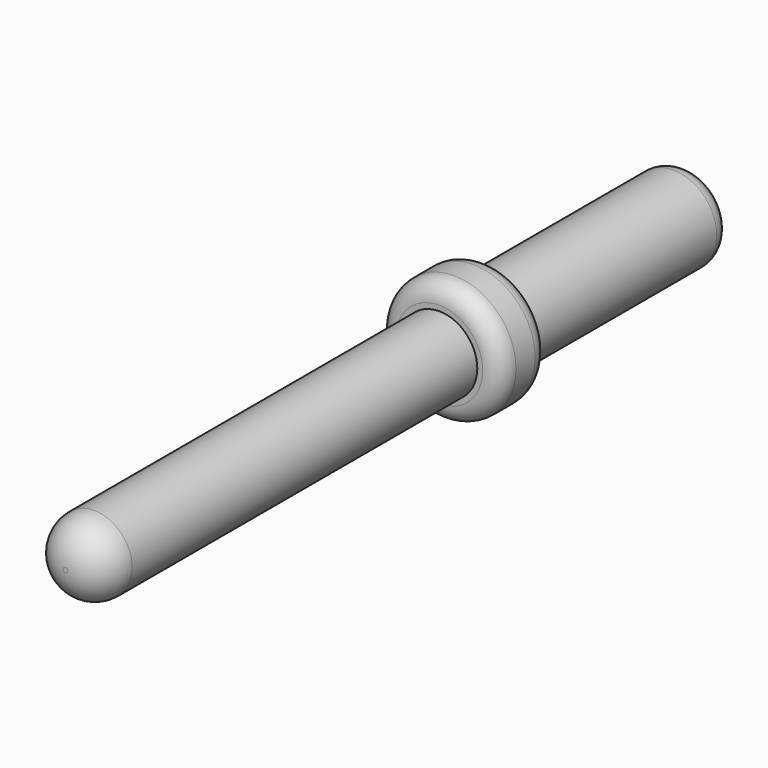
from build123d import *

# Parameters (mm, degrees)
F0_R     = 10.4764033566
F1_DEPTH = 128.524
F2_R     = 9.8113639175
F3_R     = 17.037591744
F4_DEPTH = 16.764
F5_R     = 5.08
F6_R     = 5.08
F7_DEPTH = 68.834
F8_R     = 5.08


with BuildPart() as f1:
    # F0 (on Front) → F1 (new body)
    with BuildSketch(Plane.XZ):
        Circle(F0_R)
    extrude(amount=F1_DEPTH)

    # F2
    f2_edges = [f1.edges().sort_by_distance(p)[0] for p in [
        (-10.476403, -128.524, 0),
    ]]
    fillet(f2_edges, radius=F2_R)

    # F3 (on Front) → F4 (join)
    with BuildSketch(Plane.XZ):
        Circle(F3_R)
    extrude(amount=-F4_DEPTH)

    # F5
    f5_edges = [f1.edges().sort_by_distance(p)[0] for p in [
        (-17.037592, 16.764, 0),
    ]]
    fillet(f5_edges, radius=F5_R)

    # F6
    f6_edges = [f1.edges().sort_by_distance(p)[0] for p in [
        (-17.037592, 0, 0),
    ]]
    fillet(f6_edges, radius=F6_R)

    # F7 (add): a face of the model
    f7_faces = [f1.faces().sort_by_distance(p)[0] for p in [
        (0, 16.764, 0),
    ]]
    extrude(f7_faces, amount=F7_DEPTH)

    # F8
    f8_edges = [f1.edges().sort_by_distance(p)[0] for p in [
        (-11.957592, 85.598, 0),
    ]]
    fillet(f8_edges, radius=F8_R)


solid = f1.part
